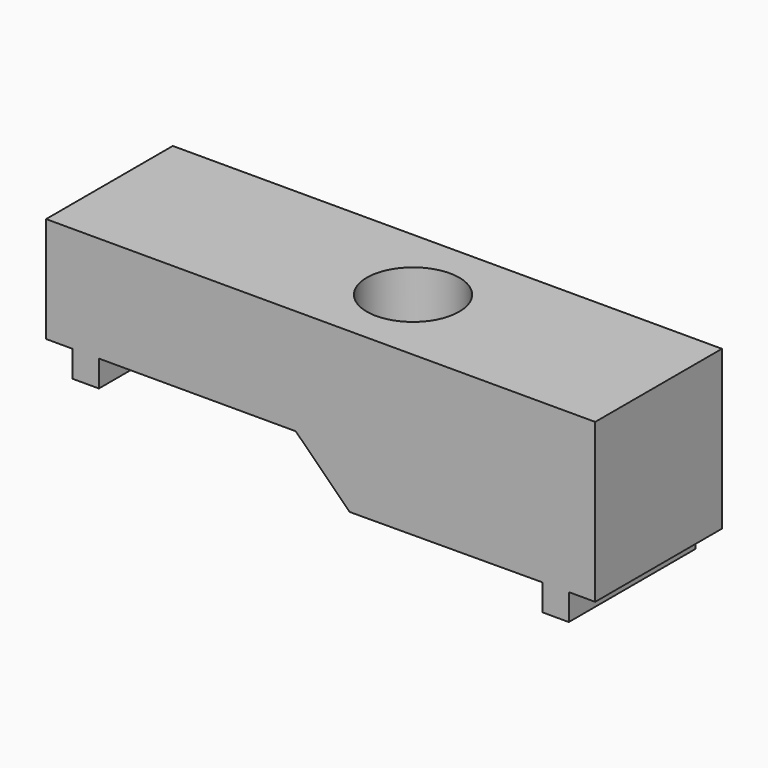
from build123d import *

# Parameters (mm, degrees)
F1_DEPTH      = 6
F2_R          = 1.75
F3_DEPTH      = 4.001
F3_DEPTH_BACK = 3.001


# Not quite as in the source:
# - a feature of the source that left no trace in its solid (it failed there, or was rolled back) is left out


with BuildPart() as f1:
    # F0 (on Front) → F1 (new body)
    with BuildSketch(Plane.XZ):
        Polygon((20.8, 0), (0, 0), (0, -4), (1, -4), (1, -5), (2, -5), (2, -4), (9.4564415496, -4), (11.5, -6.0279625468), (18.8, -6), (18.8, -7), (19.8, -7), (19.8, -6), (20.8, -6), align=None)
    extrude(amount=F1_DEPTH)

    # F2 (on face) → F3 (cut, two sides)
    with BuildSketch(Plane(origin=(0, 0, -4), x_dir=(1, 0, 0), z_dir=(0, 0, -1))) as f3_sk:
        with Locations((11.5, 3)):
            Circle(F2_R)
    extrude(amount=-F3_DEPTH, mode=Mode.SUBTRACT)
    extrude(f3_sk.sketch, amount=F3_DEPTH_BACK, mode=Mode.SUBTRACT)


solid = f1.part
